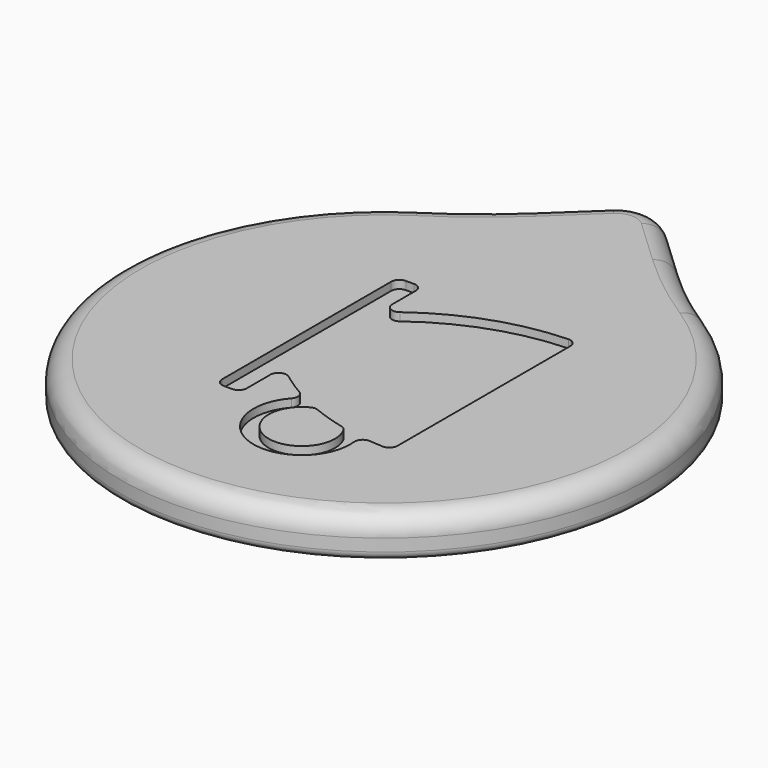
from build123d import *

# Parameters (mm, degrees)
F1_DEPTH = 10
F2_R     = 10
F3_R     = 120
F4_T     = -5
F5_R     = 5
F7_DEPTH = 2
F8_R     = 2
F9_R     = 2


with BuildPart() as f1:
    # F0 (on Top) → F1 (new body)
    with BuildSketch(Plane.XY):
        with BuildLine():
            Line((0, 85), (-28, 58.6600375042))
            ThreePointArc((-28, 58.6600375042), (0, -65), (28, 58.6600375042))
            Line((28, 58.6600375042), (0, 85))
        make_face()
    extrude(amount=F1_DEPTH)

    # F2
    f2_edges = [f1.edges().sort_by_distance(p)[0] for p in [
        (0, 85, 5),
    ]]
    fillet(f2_edges, radius=F2_R)

    # F3
    f3_edges = [f1.edges().sort_by_distance(p)[0] for p in [
        (-28, 58.660038, 5),
        (28, 58.660038, 5),
    ]]
    fillet(f3_edges, radius=F3_R)

    # F4
    f4_openings = [f1.faces().sort_by_distance(p)[0] for p in [
        (0, 2.490227, 0),
    ]]
    offset(amount=F4_T, openings=f4_openings)

    # F5
    f5_edges = [f1.edges().sort_by_distance(p)[0] for p in [
        (0, -65, 10),
        (12.376367, 73.357391, 10),
        (26.230576, 61.013655, 10),
        (0, 81.270685, 10),
        (-12.376367, 73.357391, 10),
        (-26.230576, 61.013655, 10),
    ]]
    fillet(f5_edges, radius=F5_R)

    # F6 (on face) → F7 (cut)
    with BuildSketch(Plane.XY.offset(10)):
        with BuildLine():
            Line((24.5830141958, -28.6241205137), (24.5830141958, 28.6241205137))
            ThreePointArc((24.5830141958, 28.6241205137), (4.5140931022, 24.9911712124), (-13.0076974051, 14.5534141782))
            Line((-13.0076974051, 14.5534141782), (-13.0076974051, 28))
            Line((-13.0076974051, 28), (-19.0571866046, 28))
            Line((-19.0571866046, 28), (-19.0571866046, -28))
            Line((-19.0571866046, -28), (-13.0076974051, -28))
            Line((-13.0076974051, -28), (-13.0076974051, -14.5534141782))
            ThreePointArc((-13.0076974051, -14.5534141782), (-7.6208581173, -18.7073881119), (-1.7793276831, -22.1930816072))
            ThreePointArc((-1.7793276831, -22.1930816072), (1.5769915618, -43.1576186172), (16.4944786534, -28.0498302354))
            ThreePointArc((16.4944786534, -28.0498302354), (20.5285655112, -28.4803674588), (24.5830141958, -28.6241205137))
        make_face()
        with BuildLine():
            ThreePointArc((11.9329452437, -27.2089956114), (2.7197472284, -39.5920744788), (2.4211464703, -24.1604673852))
            ThreePointArc((2.4211464703, -24.1604673852), (7.1104323918, -25.8925740471), (11.9329452437, -27.2089956114))
        make_face(mode=Mode.SUBTRACT)
    extrude(amount=-F7_DEPTH, mode=Mode.SUBTRACT)

    # F8
    f8_edges = [f1.edges().sort_by_distance(p)[0] for p in [
        (-13.007697, 28, 9),
        (-19.057187, 28, 9),
        (-13.007697, 14.553414, 9),
        (24.583014, 28.624121, 9),
        (24.583014, -28.624121, 9),
        (16.494479, -28.04983, 9),
        (-1.779328, -22.193082, 9),
        (2.421146, -24.160467, 9),
        (11.932945, -27.208996, 9),
        (-13.007697, -14.553414, 9),
        (-13.007697, -28, 9),
        (-19.057187, -28, 9),
    ]]
    fillet(f8_edges, radius=F8_R)

    # F9
    f9_edges = [f1.edges().sort_by_distance(p)[0] for p in [
        (0, -65, 0),
        (-26.230576, 61.013655, 0),
        (26.230576, 61.013655, 0),
        (-12.376367, 73.357391, 0),
        (12.376367, 73.357391, 0),
        (0, 81.270685, 0),
        (8.950439, 69.715549, 0),
        (23.151719, 57.074031, 0),
        (0, -60, 0),
        (-23.151719, 57.074031, 0),
        (-8.950439, 69.715549, 0),
        (0, 76.270685, 0),
    ]]
    fillet(f9_edges, radius=F9_R)


solid = f1.part
